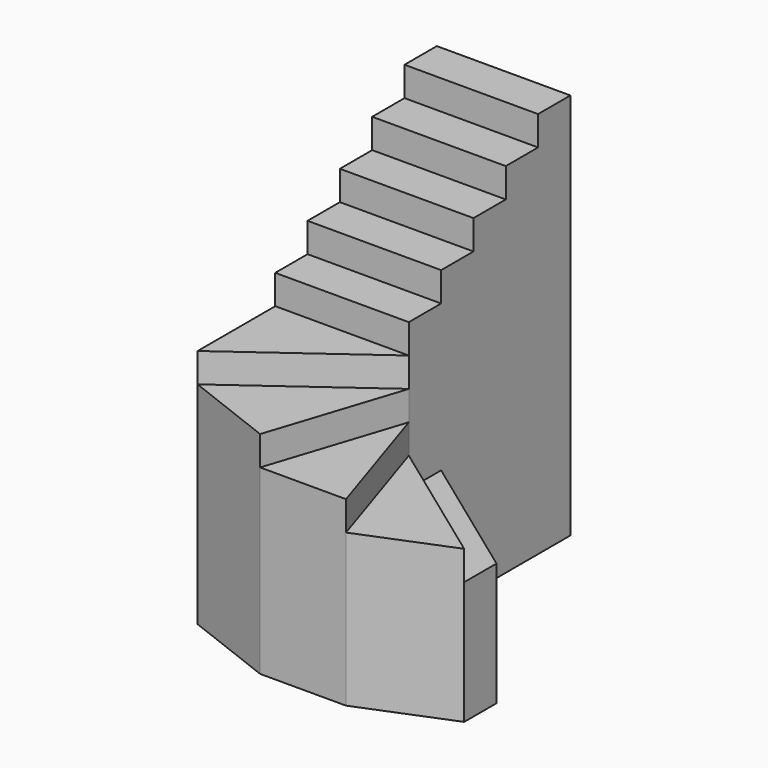
from build123d import *

# Parameters (mm, degrees)
F0_W      = 923.925
F0_H      = 279.4
F1_DEPTH  = 2679.7
F2_W      = 923.925
F2_H      = 279.4
F3_DEPTH  = 2476.5
F4_W      = 923.925
F4_H      = 279.4
F5_DEPTH  = 2273.3
F6_W      = 923.925
F6_H      = 279.4
F7_DEPTH  = 2070.1
F8_W      = 923.925
F8_H      = 279.4
F9_DEPTH  = 1866.9
F11_DEPTH = 1663.7
F13_DEPTH = 1460.5
F15_DEPTH = 1257.3
F18_DEPTH = 1054.1
F20_DEPTH = 850.9


with BuildPart() as f1:
    # F0 (on Top) → F1 (new body)
    with BuildSketch(Plane.XY):
        with Locations((461.9625, -139.7)):
            Rectangle(F0_W, F0_H)
    extrude(amount=F1_DEPTH)

    # F2 (on face) → F3 (join)
    with BuildSketch(Plane(origin=(0, 0, 0), x_dir=(1, 0, 0), z_dir=(0, 0, -1))):
        with Locations((461.9625, 419.1)):
            Rectangle(F2_W, F2_H)
    extrude(amount=-F3_DEPTH)

    # F4 (on face) → F5 (join)
    with BuildSketch(Plane(origin=(0, 0, 0), x_dir=(1, 0, 0), z_dir=(0, 0, -1))):
        with Locations((461.9625, 698.5)):
            Rectangle(F4_W, F4_H)
    extrude(amount=-F5_DEPTH)

    # F6 (on face) → F7 (join)
    with BuildSketch(Plane(origin=(0, 0, 0), x_dir=(1, 0, 0), z_dir=(0, 0, -1))):
        with Locations((461.9625, 977.9)):
            Rectangle(F6_W, F6_H)
    extrude(amount=-F7_DEPTH)

    # F8 (on face) → F9 (join)
    with BuildSketch(Plane(origin=(0, 0, 0), x_dir=(1, 0, 0), z_dir=(0, 0, -1))):
        with Locations((461.9625, 1257.3)):
            Rectangle(F8_W, F8_H)
    extrude(amount=-F9_DEPTH)


with BuildPart() as f11:
    # F10 (on face) → F11 (new body)
    with BuildSketch(Plane(origin=(0, 0, 0), x_dir=(1, 0, 0), z_dir=(0, 0, -1))):
        Polygon((0, 1397), (923.925, 1397), (0, 2068.2708051874), align=None)
    extrude(amount=-F11_DEPTH)

    # F12 (on face) → F13 (join)
    with BuildSketch(Plane(origin=(0, 0, 0), x_dir=(1, 0, 0), z_dir=(0, 0, -1))):
        Polygon((0, 2068.2708051874), (923.925, 1397), (626.8184297646, 2311.4), align=None)
    extrude(amount=-F13_DEPTH)

    # F14 (on face) → F15 (join)
    with BuildSketch(Plane(origin=(0, 0, 0), x_dir=(1, 0, 0), z_dir=(0, 0, -1))):
        Polygon((626.8184297646, 2311.4), (923.925, 1397), (1221.0315702354, 2311.4), align=None)
    extrude(amount=-F15_DEPTH)

    # F17 (on face) → F18 (join)
    with BuildSketch(Plane(origin=(0, 0, 0), x_dir=(1, 0, 0), z_dir=(0, 0, -1))):
        Polygon((1221.0315702354, 2311.4), (923.925, 1397), (1838.325, 2061.3504876081), align=None)
    extrude(amount=-F18_DEPTH)


with BuildPart() as f20:
    # F19 (on face) → F20 (new body)
    with BuildSketch(Plane(origin=(0, 0, 0), x_dir=(1, 0, 0), z_dir=(0, 0, -1))):
        Polygon((1838.325, 1781.9504876081), (1838.325, 2061.3504876081), (923.925, 1397), (923.925, 1117.6), align=None)
    extrude(amount=-F20_DEPTH)


solid = Compound([f1.part, f11.part, f20.part])
